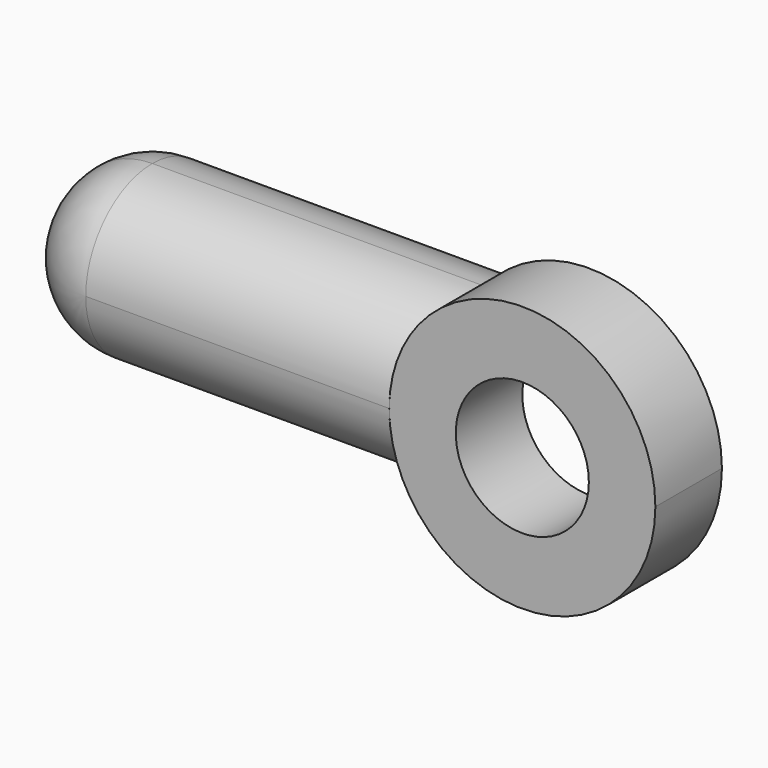
from build123d import *

# Parameters (mm, degrees)
F1_DEPTH = 6.35
F2_R     = 6.3499
F0_R     = 5.08
F3_DEPTH = 6.35


# Not quite as in the source:
# - a fillet or chamfer is up to 0.001 mm smaller than in the source, because OpenCascade refuses the exact size


with BuildPart() as f1:
    # F0 (on Front) → F1 (new body, symmetric)
    with BuildSketch(Plane.XZ):
        with BuildLine():
            Line((12.7, 6.35), (-12.7, 6.35))
            Line((-12.7, 6.35), (-12.7, -6.35))
            Line((-12.7, -6.35), (12.7, -6.35))
            ThreePointArc((12.7, -6.35), (10.471147458, 0), (12.7, 6.35))
        make_face()
        with BuildLine():
            Line((-12.7, -6.35), (-12.7, 6.35))
            ThreePointArc((-12.7, 6.35), (-19.05, 0), (-12.7, -6.35))
        make_face()
    extrude(amount=F1_DEPTH, both=True)

    # F2 (radius 6.35 in the source; OpenCascade refuses exactly that, so slightly less here)
    f2_edges = [f1.edges().sort_by_distance(p)[0] for p in [
        (0, -6.35, 6.35),
        (0, 6.35, 6.35),
        (0, -6.35, -6.35),
        (0, 6.35, -6.35),
    ]]
    fillet(f2_edges, radius=F2_R)

    # F0 (on Front) → F3 (join)
    with BuildSketch(Plane.XZ):
        with BuildLine():
            ThreePointArc((30.791147458, 0), (23.9960502669, 9.5866067556), (12.7, 6.35))
            Line((12.7, 6.35), (12.7, -6.35))
            ThreePointArc((12.7, -6.35), (23.9960502669, -9.5866067556), (30.791147458, 0))
        make_face()
        with Locations((20.631147458, 0)):
            Circle(F0_R, mode=Mode.SUBTRACT)
        with BuildLine():
            Line((12.7, -6.35), (12.7, 6.35))
            ThreePointArc((12.7, 6.35), (10.471147458, 0), (12.7, -6.35))
        make_face()
    extrude(amount=F3_DEPTH)


solid = f1.part
